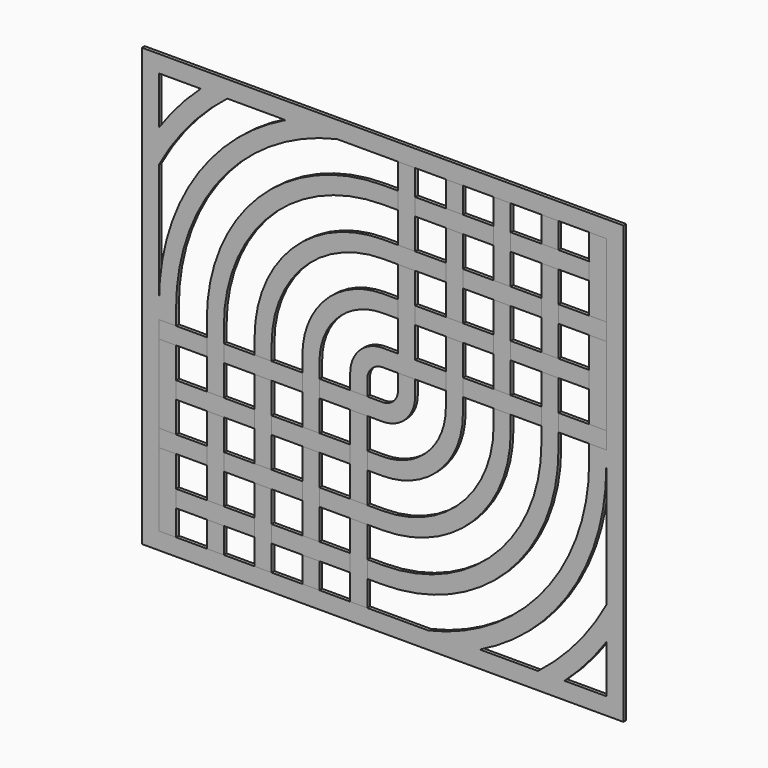
from build123d import *

# Parameters (mm, degrees)
F1_DEPTH  = 6.35
F2_DEPTH  = 6.35
F3_DEPTH  = 6.35
F4_DEPTH  = 6.35
F0_W      = 31.75
F0_H      = 47.625
F5_DEPTH  = 6.35
F6_DEPTH  = 6.35
F7_DEPTH  = 6.35
F8_DEPTH  = 6.35
F9_DEPTH  = 6.35
F10_DEPTH = 6.35


with BuildPart() as f1:
    # F0 (on Front) → F1 (new body)
    with BuildSketch(Plane.XZ):
        Polygon((-447.675, -406.4), (447.675, -406.4), (447.675, 0), (447.675, 406.4), (-447.675, 406.4), (-447.675, 0), align=None)
        Polygon((28.575, 374.65), (60.325, 374.65), (117.475, 374.65), (149.225, 374.65), (206.375, 374.65), (238.125, 374.65), (295.275, 374.65), (327.025, 374.65), (384.175, 374.65), (415.925, 374.65), (415.925, 238.125), (415.925, 206.375), (415.925, 60.325), (415.925, 28.575), (415.925, 0), (415.925, -225.4026397361), (415.925, -286.1025602821), (415.925, -374.65), (338.3572935892, -374.65), (288.8552113516, -374.65), (180.6404803055, -374.65), (85.0165167776, -374.65), (-28.575, -374.65), (-60.325, -374.65), (-117.475, -374.65), (-149.225, -374.65), (-206.375, -374.65), (-238.125, -374.65), (-295.275, -374.65), (-327.025, -374.65), (-384.175, -374.65), (-415.925, -374.65), (-415.925, -238.125), (-415.925, -206.375), (-415.925, -60.325), (-415.925, -28.575), (-415.925, 0), (-415.925, 225.4026397361), (-415.925, 286.1025602821), (-415.925, 374.65), (-338.3572935892, 374.65), (-288.8552113516, 374.65), (-180.6404803055, 374.65), (-85.0165167776, 374.65), align=None, mode=Mode.SUBTRACT)
    extrude(amount=F1_DEPTH)

    # F0 (on Front) → F2, piece 6 (join)
    with BuildSketch(Plane.XZ):
        with BuildLine():
            Line((-415.925, 286.1025602821), (-415.925, 225.4026397361))
            ThreePointArc((-415.925, 225.4026397361), (-360.2047753912, 306.6797603533), (-288.8552113516, 374.65))
            Line((-288.8552113516, 374.65), (-338.3572935892, 374.65))
            ThreePointArc((-338.3572935892, 374.65), (-379.7309664429, 332.6449665173), (-415.925, 286.1025602821))
        make_face()
        with BuildLine():
            Line((-415.925, -28.575), (-384.175, -28.575))
            Line((-384.175, -28.575), (-384.175, 0))
            ThreePointArc((-384.175, 0), (-300.2096358864, 239.717761432), (-85.0165167776, 374.65))
            Line((-85.0165167776, 374.65), (-180.6404803055, 374.65))
            ThreePointArc((-180.6404803055, 374.65), (-352.2261329005, 221.20207261), (-415.925, 0))
            Line((-415.925, 0), (-415.925, -28.575))
        make_face()
        with BuildLine():
            Line((415.925, 28.575), (384.175, 28.575))
            Line((384.175, 28.575), (384.175, 0))
            ThreePointArc((384.175, 0), (300.2096358864, -239.717761432), (85.0165167776, -374.65))
            Line((85.0165167776, -374.65), (180.6404803055, -374.65))
            ThreePointArc((180.6404803055, -374.65), (352.2261329005, -221.20207261), (415.925, 0))
            Line((415.925, 0), (415.925, 28.575))
        make_face()
        with BuildLine():
            Line((415.925, -286.1025602821), (415.925, -225.4026397361))
            ThreePointArc((415.925, -225.4026397361), (360.2047753912, -306.6797603533), (288.8552113516, -374.65))
            Line((288.8552113516, -374.65), (338.3572935892, -374.65))
            ThreePointArc((338.3572935892, -374.65), (379.7309664429, -332.6449665173), (415.925, -286.1025602821))
        make_face()
    extrude(amount=F2_DEPTH)


with BuildPart() as f2:
    # F0 (on Front) → F2 (new body)
    with BuildSketch(Plane.XZ):
        with BuildLine():
            Line((-295.275, -117.475), (-295.275, -60.325))
            Line((-295.275, -60.325), (-295.275, -28.575))
            Line((-295.275, -28.575), (-295.275, 0))
            ThreePointArc((-295.275, 0), (-208.7909548149, 208.7909548149), (0, 295.275))
            Line((0, 295.275), (28.575, 295.275))
            Line((28.575, 295.275), (28.575, 327.025))
            Line((28.575, 327.025), (0, 327.025))
            ThreePointArc((0, 327.025), (-231.2415951175, 231.2415951175), (-327.025, 0))
            Line((-327.025, 0), (-327.025, -28.575))
            Line((-327.025, -28.575), (-327.025, -60.325))
            Line((-327.025, -60.325), (-327.025, -117.475))
            Line((-327.025, -117.475), (-295.275, -117.475))
        make_face()
    extrude(amount=F2_DEPTH)


with BuildPart() as f2b:
    # F0 (on Front) → F2, piece 2 (new body)
    with BuildSketch(Plane.XZ):
        with BuildLine():
            Line((28.575, 206.375), (60.325, 206.375))
            Line((60.325, 206.375), (117.475, 206.375))
            Line((117.475, 206.375), (117.475, 207.1307316648))
            Line((117.475, 207.1307316648), (117.475, 238.125))
            Line((117.475, 238.125), (60.325, 238.125))
            Line((60.325, 238.125), (28.575, 238.125))
            Line((28.575, 238.125), (0, 238.125))
            ThreePointArc((0, 238.125), (-168.37980227, 168.37980227), (-238.125, 0))
            Line((-238.125, 0), (-238.125, -28.575))
            Line((-238.125, -28.575), (-206.375, -28.575))
            Line((-206.375, -28.575), (-206.375, 0))
            ThreePointArc((-206.375, 0), (-145.9291619674, 145.9291619674), (0, 206.375))
            Line((0, 206.375), (28.575, 206.375))
        make_face()
    extrude(amount=F2_DEPTH)


with BuildPart() as f2c:
    # F0 (on Front) → F2, piece 3 (new body)
    with BuildSketch(Plane.XZ):
        with BuildLine():
            Line((-117.475, -60.325), (-117.475, -28.575))
            Line((-117.475, -28.575), (-117.475, 0))
            ThreePointArc((-117.475, 0), (-83.0673691199, 83.0673691199), (0, 117.475))
            Line((0, 117.475), (28.575, 117.475))
            Line((28.575, 117.475), (28.575, 149.225))
            Line((28.575, 149.225), (0, 149.225))
            ThreePointArc((0, 149.225), (-105.5180094226, 105.5180094226), (-149.225, 0))
            Line((-149.225, 0), (-149.225, -28.575))
            Line((-149.225, -28.575), (-149.225, -60.325))
            Line((-149.225, -60.325), (-149.225, -117.475))
            Line((-149.225, -117.475), (-117.475, -117.475))
            Line((-117.475, -117.475), (-117.475, -60.325))
        make_face()
        with BuildLine():
            ThreePointArc((-28.575, 0), (-20.2055762724, 20.2055762724), (0, 28.575))
            Line((0, 28.575), (28.575, 28.575))
            Line((28.575, 28.575), (60.325, 28.575))
            Line((60.325, 28.575), (117.475, 28.575))
            Line((117.475, 28.575), (117.475, 60.325))
            Line((117.475, 60.325), (60.325, 60.325))
            Line((60.325, 60.325), (28.575, 60.325))
            Line((28.575, 60.325), (0, 60.325))
            ThreePointArc((0, 60.325), (-42.6562165751, 42.6562165751), (-60.325, 0))
            Line((-60.325, 0), (-60.325, -28.575))
            Line((-60.325, -28.575), (-28.575, -28.575))
            Line((-28.575, -28.575), (-28.575, 0))
        make_face()
        with BuildLine():
            Line((60.325, 28.575), (28.575, 28.575))
            Line((28.575, 28.575), (28.575, 0))
            ThreePointArc((28.575, 0), (20.2055762724, -20.2055762724), (0, -28.575))
            Line((0, -28.575), (-28.575, -28.575))
            Line((-28.575, -28.575), (-60.325, -28.575))
            Line((-60.325, -28.575), (-117.475, -28.575))
            Line((-117.475, -28.575), (-117.475, -60.325))
            Line((-117.475, -60.325), (-60.325, -60.325))
            Line((-60.325, -60.325), (-28.575, -60.325))
            Line((-28.575, -60.325), (0, -60.325))
            ThreePointArc((0, -60.325), (42.6562165751, -42.6562165751), (60.325, 0))
            Line((60.325, 0), (60.325, 28.575))
        make_face()
        with BuildLine():
            Line((117.475, 60.325), (117.475, 28.575))
            Line((117.475, 28.575), (117.475, 0))
            ThreePointArc((117.475, 0), (83.0673691199, -83.0673691199), (0, -117.475))
            Line((0, -117.475), (-28.575, -117.475))
            Line((-28.575, -117.475), (-28.575, -149.225))
            Line((-28.575, -149.225), (0, -149.225))
            ThreePointArc((0, -149.225), (105.5180094226, -105.5180094226), (149.225, 0))
            Line((149.225, 0), (149.225, 28.575))
            Line((149.225, 28.575), (149.225, 60.325))
            Line((149.225, 60.325), (149.225, 117.475))
            Line((149.225, 117.475), (117.475, 117.475))
            Line((117.475, 117.475), (117.475, 60.325))
        make_face()
    extrude(amount=F2_DEPTH)


with BuildPart() as f2d:
    # F0 (on Front) → F2, piece 4 (new body)
    with BuildSketch(Plane.XZ):
        with BuildLine():
            Line((0, -206.375), (-28.575, -206.375))
            Line((-28.575, -206.375), (-60.325, -206.375))
            Line((-60.325, -206.375), (-117.475, -206.375))
            Line((-117.475, -206.375), (-118.7976220301, -206.375))
            ThreePointArc((-118.7976220301, -206.375), (-118.1369153264, -206.7539234505), (-117.475, -207.1307316648))
            Line((-117.475, -207.1307316648), (-117.475, -238.125))
            Line((-117.475, -238.125), (-60.325, -238.125))
            Line((-60.325, -238.125), (-28.575, -238.125))
            Line((-28.575, -238.125), (0, -238.125))
            ThreePointArc((0, -238.125), (168.37980227, -168.37980227), (238.125, 0))
            Line((238.125, 0), (238.125, 28.575))
            Line((238.125, 28.575), (206.375, 28.575))
            Line((206.375, 28.575), (206.375, 0))
            ThreePointArc((206.375, 0), (145.9291619674, -145.9291619674), (0, -206.375))
        make_face()
    extrude(amount=F2_DEPTH)


with BuildPart() as f2e:
    # F0 (on Front) → F2, piece 5 (new body)
    with BuildSketch(Plane.XZ):
        with BuildLine():
            Line((295.275, 117.475), (295.275, 60.325))
            Line((295.275, 60.325), (295.275, 28.575))
            Line((295.275, 28.575), (295.275, 0))
            ThreePointArc((295.275, 0), (208.7909548149, -208.7909548149), (0, -295.275))
            Line((0, -295.275), (-28.575, -295.275))
            Line((-28.575, -295.275), (-28.575, -327.025))
            Line((-28.575, -327.025), (0, -327.025))
            ThreePointArc((0, -327.025), (231.2415951175, -231.2415951175), (327.025, 0))
            Line((327.025, 0), (327.025, 28.575))
            Line((327.025, 28.575), (327.025, 60.325))
            Line((327.025, 60.325), (327.025, 117.475))
            Line((327.025, 117.475), (295.275, 117.475))
        make_face()
    extrude(amount=F2_DEPTH)


with BuildPart() as f3:
    # F0 (on Front) → F3 (new body)
    with BuildSketch(Plane.XZ):
        Polygon((-384.175, -60.325), (-327.025, -60.325), (-327.025, -28.575), (-384.175, -28.575), (-415.925, -28.575), (-415.925, -60.325), align=None)
    extrude(amount=F3_DEPTH)


with BuildPart() as f3b:
    # F0 (on Front) → F3, piece 2 (new body)
    with BuildSketch(Plane.XZ):
        Polygon((-206.375, -60.325), (-149.225, -60.325), (-149.225, -28.575), (-206.375, -28.575), (-238.125, -28.575), (-295.275, -28.575), (-295.275, -60.325), (-238.125, -60.325), align=None)
    extrude(amount=F3_DEPTH)


with BuildPart() as f3c:
    # F0 (on Front) → F3, piece 3 (new body)
    with BuildSketch(Plane.XZ):
        Polygon((-238.125, -149.225), (-238.125, -117.475), (-295.275, -117.475), (-327.025, -117.475), (-384.175, -117.475), (-384.175, -149.225), (-327.025, -149.225), (-295.275, -149.225), align=None)
    extrude(amount=F3_DEPTH)


with BuildPart() as f3d:
    # F0 (on Front) → F3, piece 4 (new body)
    with BuildSketch(Plane.XZ):
        Polygon((-60.325, -117.475), (-117.475, -117.475), (-149.225, -117.475), (-206.375, -117.475), (-206.375, -149.225), (-149.225, -149.225), (-117.475, -149.225), (-60.325, -149.225), align=None)
    extrude(amount=F3_DEPTH)


with BuildPart() as f3e:
    # F0 (on Front) → F3, piece 5 (new body)
    with BuildSketch(Plane.XZ):
        Polygon((-327.025, -238.125), (-327.025, -206.375), (-384.175, -206.375), (-415.925, -206.375), (-415.925, -238.125), (-384.175, -238.125), align=None)
    extrude(amount=F3_DEPTH)


with BuildPart() as f3f:
    # F0 (on Front) → F3, piece 6 (new body)
    with BuildSketch(Plane.XZ):
        Polygon((-149.225, -206.375), (-206.375, -206.375), (-238.125, -206.375), (-295.275, -206.375), (-295.275, -238.125), (-238.125, -238.125), (-206.375, -238.125), (-149.225, -238.125), align=None)
    extrude(amount=F3_DEPTH)


with BuildPart() as f3g:
    # F0 (on Front) → F3, piece 7 (new body)
    with BuildSketch(Plane.XZ):
        Polygon((-238.125, -295.275), (-295.275, -295.275), (-327.025, -295.275), (-384.175, -295.275), (-384.175, -327.025), (-327.025, -327.025), (-295.275, -327.025), (-238.125, -327.025), align=None)
    extrude(amount=F3_DEPTH)


with BuildPart() as f3h:
    # F0 (on Front) → F3, piece 8 (new body)
    with BuildSketch(Plane.XZ):
        Polygon((-117.475, -295.275), (-149.225, -295.275), (-206.375, -295.275), (-206.375, -327.025), (-149.225, -327.025), (-117.475, -327.025), (-60.325, -327.025), (-60.325, -295.275), align=None)
    extrude(amount=F3_DEPTH)


with BuildPart() as f4:
    # F0 (on Front) → F4 (new body)
    with BuildSketch(Plane.XZ):
        Polygon((-384.175, -149.225), (-384.175, -117.475), (-384.175, -60.325), (-415.925, -60.325), (-415.925, -206.375), (-384.175, -206.375), align=None)
    extrude(amount=F4_DEPTH)


with BuildPart() as f4b:
    # F0 (on Front) → F4, piece 2 (new body)
    with BuildSketch(Plane.XZ):
        Polygon((-295.275, -238.125), (-295.275, -206.375), (-295.275, -149.225), (-327.025, -149.225), (-327.025, -206.375), (-327.025, -238.125), (-327.025, -295.275), (-295.275, -295.275), align=None)
    extrude(amount=F4_DEPTH)


with BuildPart() as f4c:
    # F0 (on Front) → F4, piece 3 (new body)
    with BuildSketch(Plane.XZ):
        Polygon((-206.375, -149.225), (-206.375, -117.475), (-206.375, -60.325), (-238.125, -60.325), (-238.125, -117.475), (-238.125, -149.225), (-238.125, -206.375), (-206.375, -206.375), align=None)
    extrude(amount=F4_DEPTH)


with BuildPart() as f4d:
    # F0 (on Front) → F4, piece 4 (new body)
    with BuildSketch(Plane.XZ):
        with BuildLine():
            Line((-117.475, -206.375), (-117.475, -149.225))
            Line((-117.475, -149.225), (-149.225, -149.225))
            Line((-149.225, -149.225), (-149.225, -206.375))
            Line((-149.225, -206.375), (-149.225, -238.125))
            Line((-149.225, -238.125), (-149.225, -295.275))
            Line((-149.225, -295.275), (-117.475, -295.275))
            Line((-117.475, -295.275), (-117.475, -238.125))
            Line((-117.475, -238.125), (-117.475, -207.1307316648))
            ThreePointArc((-117.475, -207.1307316648), (-118.1369153264, -206.7539234505), (-118.7976220301, -206.375))
            Line((-118.7976220301, -206.375), (-117.475, -206.375))
        make_face()
    extrude(amount=F4_DEPTH)


with BuildPart() as f4e:
    # F0 (on Front) → F4, piece 5 (new body)
    with BuildSketch(Plane.XZ):
        Polygon((-206.375, -295.275), (-206.375, -238.125), (-238.125, -238.125), (-238.125, -295.275), (-238.125, -327.025), (-238.125, -374.65), (-206.375, -374.65), (-206.375, -327.025), align=None)
    extrude(amount=F4_DEPTH)


with BuildPart() as f4f:
    # F0 (on Front) → F4, piece 6 (new body)
    with BuildSketch(Plane.XZ):
        Polygon((-28.575, -117.475), (-28.575, -60.325), (-60.325, -60.325), (-60.325, -117.475), (-60.325, -149.225), (-60.325, -206.375), (-28.575, -206.375), (-28.575, -149.225), align=None)
    extrude(amount=F4_DEPTH)


with BuildPart() as f4g:
    # F0 (on Front) → F4, piece 7 (new body)
    with BuildSketch(Plane.XZ):
        Polygon((-28.575, -295.275), (-28.575, -238.125), (-60.325, -238.125), (-60.325, -295.275), (-60.325, -327.025), (-60.325, -374.65), (-28.575, -374.65), (-28.575, -327.025), align=None)
    extrude(amount=F4_DEPTH)


with BuildPart() as f4h:
    # F0 (on Front) → F4, piece 8 (new body)
    with BuildSketch(Plane.XZ):
        with Locations((-133.35, -350.8375)):
            Rectangle(F0_W, F0_H)
    extrude(amount=F4_DEPTH)


with BuildPart() as f4i:
    # F0 (on Front) → F4, piece 9 (new body)
    with BuildSketch(Plane.XZ):
        with Locations((-311.15, -350.8375)):
            Rectangle(F0_W, F0_H)
    extrude(amount=F4_DEPTH)


with BuildPart() as f4j:
    # F0 (on Front) → F4, piece 10 (new body)
    with BuildSketch(Plane.XZ):
        with BuildLine():
            Line((-384.175, -327.025), (-384.175, -295.275))
            Line((-384.175, -295.275), (-384.175, -238.125))
            Line((-384.175, -238.125), (-415.925, -238.125))
            Line((-415.925, -238.125), (-415.925, -374.65))
            Line((-415.925, -374.65), (-384.175, -374.65))
            Line((-384.175, -374.65), (-384.175, -327.502442739))
            ThreePointArc((-384.175, -327.502442739), (-384.3783240375, -327.2637844845), (-384.5814998151, -327.025))
            Line((-384.5814998151, -327.025), (-384.175, -327.025))
        make_face()
    extrude(amount=F4_DEPTH)


with BuildPart() as f5:
    # F0 (on Front) → F5 (new body)
    with BuildSketch(Plane.XZ):
        Polygon((28.575, 238.125), (60.325, 238.125), (60.325, 295.275), (60.325, 327.025), (60.325, 374.65), (28.575, 374.65), (28.575, 327.025), (28.575, 295.275), align=None)
    extrude(amount=F5_DEPTH)


with BuildPart() as f5b:
    # F0 (on Front) → F5, piece 2 (new body)
    with BuildSketch(Plane.XZ):
        with Locations((133.35, 350.8375)):
            Rectangle(F0_W, F0_H)
    extrude(amount=F5_DEPTH)


with BuildPart() as f5c:
    # F0 (on Front) → F5, piece 3 (new body)
    with BuildSketch(Plane.XZ):
        with BuildLine():
            Line((117.475, 206.375), (117.475, 149.225))
            Line((117.475, 149.225), (149.225, 149.225))
            Line((149.225, 149.225), (149.225, 206.375))
            Line((149.225, 206.375), (149.225, 238.125))
            Line((149.225, 238.125), (149.225, 295.275))
            Line((149.225, 295.275), (117.475, 295.275))
            Line((117.475, 295.275), (117.475, 238.125))
            Line((117.475, 238.125), (117.475, 207.1307316648))
            ThreePointArc((117.475, 207.1307316648), (118.1369153264, 206.7539234505), (118.7976220301, 206.375))
            Line((118.7976220301, 206.375), (117.475, 206.375))
        make_face()
    extrude(amount=F5_DEPTH)


with BuildPart() as f5d:
    # F0 (on Front) → F5, piece 4 (new body)
    with BuildSketch(Plane.XZ):
        Polygon((206.375, 295.275), (206.375, 238.125), (238.125, 238.125), (238.125, 295.275), (238.125, 327.025), (238.125, 374.65), (206.375, 374.65), (206.375, 327.025), align=None)
    extrude(amount=F5_DEPTH)


with BuildPart() as f5e:
    # F0 (on Front) → F5, piece 5 (new body)
    with BuildSketch(Plane.XZ):
        with Locations((311.15, 350.8375)):
            Rectangle(F0_W, F0_H)
    extrude(amount=F5_DEPTH)


with BuildPart() as f5f:
    # F0 (on Front) → F5, piece 6 (new body)
    with BuildSketch(Plane.XZ):
        Polygon((295.275, 238.125), (295.275, 206.375), (295.275, 149.225), (327.025, 149.225), (327.025, 206.375), (327.025, 238.125), (327.025, 295.275), (295.275, 295.275), align=None)
    extrude(amount=F5_DEPTH)


with BuildPart() as f5g:
    # F0 (on Front) → F5, piece 7 (new body)
    with BuildSketch(Plane.XZ):
        with BuildLine():
            Line((384.175, 327.025), (384.175, 295.275))
            Line((384.175, 295.275), (384.175, 238.125))
            Line((384.175, 238.125), (415.925, 238.125))
            Line((415.925, 238.125), (415.925, 374.65))
            Line((415.925, 374.65), (384.175, 374.65))
            Line((384.175, 374.65), (384.175, 327.502442739))
            ThreePointArc((384.175, 327.502442739), (384.3783240375, 327.2637844845), (384.5814998151, 327.025))
            Line((384.5814998151, 327.025), (384.175, 327.025))
        make_face()
    extrude(amount=F5_DEPTH)


with BuildPart() as f5h:
    # F0 (on Front) → F5, piece 8 (new body)
    with BuildSketch(Plane.XZ):
        Polygon((384.175, 149.225), (384.175, 117.475), (384.175, 60.325), (415.925, 60.325), (415.925, 206.375), (384.175, 206.375), align=None)
    extrude(amount=F5_DEPTH)


with BuildPart() as f5i:
    # F0 (on Front) → F5, piece 9 (new body)
    with BuildSketch(Plane.XZ):
        Polygon((206.375, 149.225), (206.375, 117.475), (206.375, 60.325), (238.125, 60.325), (238.125, 117.475), (238.125, 149.225), (238.125, 206.375), (206.375, 206.375), align=None)
    extrude(amount=F5_DEPTH)


with BuildPart() as f5j:
    # F0 (on Front) → F5, piece 10 (new body)
    with BuildSketch(Plane.XZ):
        Polygon((28.575, 60.325), (60.325, 60.325), (60.325, 117.475), (60.325, 149.225), (60.325, 206.375), (28.575, 206.375), (28.575, 149.225), (28.575, 117.475), align=None)
    extrude(amount=F5_DEPTH)

    # F0 (on Front) → F8 (join)
    with BuildSketch(Plane.XZ):
        with BuildLine():
            ThreePointArc((-28.575, 0), (-20.2055762724, 20.2055762724), (0, 28.575))
            Line((0, 28.575), (28.575, 28.575))
            Line((28.575, 28.575), (60.325, 28.575))
            Line((60.325, 28.575), (117.475, 28.575))
            Line((117.475, 28.575), (117.475, 60.325))
            Line((117.475, 60.325), (60.325, 60.325))
            Line((60.325, 60.325), (28.575, 60.325))
            Line((28.575, 60.325), (0, 60.325))
            ThreePointArc((0, 60.325), (-42.6562165751, 42.6562165751), (-60.325, 0))
            Line((-60.325, 0), (-60.325, -28.575))
            Line((-60.325, -28.575), (-28.575, -28.575))
            Line((-28.575, -28.575), (-28.575, 0))
        make_face()
    extrude(amount=F8_DEPTH)


with BuildPart() as f6:
    # F0 (on Front) → F6 (new body)
    with BuildSketch(Plane.XZ):
        Polygon((60.325, 295.275), (117.475, 295.275), (149.225, 295.275), (206.375, 295.275), (206.375, 327.025), (149.225, 327.025), (117.475, 327.025), (60.325, 327.025), align=None)
    extrude(amount=F6_DEPTH)


with BuildPart() as f6b:
    # F0 (on Front) → F6, piece 2 (new body)
    with BuildSketch(Plane.XZ):
        Polygon((238.125, 295.275), (295.275, 295.275), (327.025, 295.275), (384.175, 295.275), (384.175, 327.025), (327.025, 327.025), (295.275, 327.025), (238.125, 327.025), align=None)
    extrude(amount=F6_DEPTH)


with BuildPart() as f6c:
    # F0 (on Front) → F6, piece 3 (new body)
    with BuildSketch(Plane.XZ):
        Polygon((149.225, 206.375), (206.375, 206.375), (238.125, 206.375), (295.275, 206.375), (295.275, 238.125), (238.125, 238.125), (206.375, 238.125), (149.225, 238.125), align=None)
    extrude(amount=F6_DEPTH)


with BuildPart() as f6d:
    # F0 (on Front) → F6, piece 4 (new body)
    with BuildSketch(Plane.XZ):
        Polygon((327.025, 238.125), (327.025, 206.375), (384.175, 206.375), (415.925, 206.375), (415.925, 238.125), (384.175, 238.125), align=None)
    extrude(amount=F6_DEPTH)


with BuildPart() as f6e:
    # F0 (on Front) → F6, piece 5 (new body)
    with BuildSketch(Plane.XZ):
        Polygon((238.125, 149.225), (238.125, 117.475), (295.275, 117.475), (327.025, 117.475), (384.175, 117.475), (384.175, 149.225), (327.025, 149.225), (295.275, 149.225), align=None)
    extrude(amount=F6_DEPTH)


with BuildPart() as f6f:
    # F0 (on Front) → F6, piece 6 (new body)
    with BuildSketch(Plane.XZ):
        Polygon((60.325, 117.475), (117.475, 117.475), (149.225, 117.475), (206.375, 117.475), (206.375, 149.225), (149.225, 149.225), (117.475, 149.225), (60.325, 149.225), align=None)
    extrude(amount=F6_DEPTH)


with BuildPart() as f6g:
    # F0 (on Front) → F6, piece 7 (new body)
    with BuildSketch(Plane.XZ):
        Polygon((206.375, 60.325), (149.225, 60.325), (149.225, 28.575), (206.375, 28.575), (238.125, 28.575), (295.275, 28.575), (295.275, 60.325), (238.125, 60.325), align=None)
    extrude(amount=F6_DEPTH)


with BuildPart() as f6h:
    # F0 (on Front) → F6, piece 8 (new body)
    with BuildSketch(Plane.XZ):
        Polygon((384.175, 60.325), (327.025, 60.325), (327.025, 28.575), (384.175, 28.575), (415.925, 28.575), (415.925, 60.325), align=None)
    extrude(amount=F6_DEPTH)


with BuildPart() as f7:
    # F0 (on Front) → F7 (new body)
    with BuildSketch(Plane.XZ):
        with BuildLine():
            Line((-117.475, -60.325), (-117.475, -28.575))
            Line((-117.475, -28.575), (-117.475, 0))
            ThreePointArc((-117.475, 0), (-83.0673691199, 83.0673691199), (0, 117.475))
            Line((0, 117.475), (28.575, 117.475))
            Line((28.575, 117.475), (28.575, 149.225))
            Line((28.575, 149.225), (0, 149.225))
            ThreePointArc((0, 149.225), (-105.5180094226, 105.5180094226), (-149.225, 0))
            Line((-149.225, 0), (-149.225, -28.575))
            Line((-149.225, -28.575), (-149.225, -60.325))
            Line((-149.225, -60.325), (-149.225, -117.475))
            Line((-149.225, -117.475), (-117.475, -117.475))
            Line((-117.475, -117.475), (-117.475, -60.325))
        make_face()
    extrude(amount=F7_DEPTH)


with BuildPart() as f9:
    # F0 (on Front) → F9 (new body)
    with BuildSketch(Plane.XZ):
        with BuildLine():
            Line((60.325, 28.575), (28.575, 28.575))
            Line((28.575, 28.575), (28.575, 0))
            ThreePointArc((28.575, 0), (20.2055762724, -20.2055762724), (0, -28.575))
            Line((0, -28.575), (-28.575, -28.575))
            Line((-28.575, -28.575), (-60.325, -28.575))
            Line((-60.325, -28.575), (-117.475, -28.575))
            Line((-117.475, -28.575), (-117.475, -60.325))
            Line((-117.475, -60.325), (-60.325, -60.325))
            Line((-60.325, -60.325), (-28.575, -60.325))
            Line((-28.575, -60.325), (0, -60.325))
            ThreePointArc((0, -60.325), (42.6562165751, -42.6562165751), (60.325, 0))
            Line((60.325, 0), (60.325, 28.575))
        make_face()
    extrude(amount=F9_DEPTH)


with BuildPart() as f10:
    # F0 (on Front) → F10 (new body)
    with BuildSketch(Plane.XZ):
        with BuildLine():
            Line((117.475, 60.325), (117.475, 28.575))
            Line((117.475, 28.575), (117.475, 0))
            ThreePointArc((117.475, 0), (83.0673691199, -83.0673691199), (0, -117.475))
            Line((0, -117.475), (-28.575, -117.475))
            Line((-28.575, -117.475), (-28.575, -149.225))
            Line((-28.575, -149.225), (0, -149.225))
            ThreePointArc((0, -149.225), (105.5180094226, -105.5180094226), (149.225, 0))
            Line((149.225, 0), (149.225, 28.575))
            Line((149.225, 28.575), (149.225, 60.325))
            Line((149.225, 60.325), (149.225, 117.475))
            Line((149.225, 117.475), (117.475, 117.475))
            Line((117.475, 117.475), (117.475, 60.325))
        make_face()
    extrude(amount=F10_DEPTH)


solid = Compound([f1.part, f2.part, f2b.part, f2c.part, f2d.part, f2e.part, f3.part, f3b.part, f3c.part, f3d.part, f3e.part, f3f.part, f3g.part, f3h.part, f4.part, f4b.part, f4c.part, f4d.part, f4e.part, f4f.part, f4g.part, f4h.part, f4i.part, f4j.part, f5.part, f5b.part, f5c.part, f5d.part, f5e.part, f5f.part, f5g.part, f5h.part, f5i.part, f5j.part, f6.part, f6b.part, f6c.part, f6d.part, f6e.part, f6f.part, f6g.part, f6h.part, f7.part, f9.part, f10.part])
